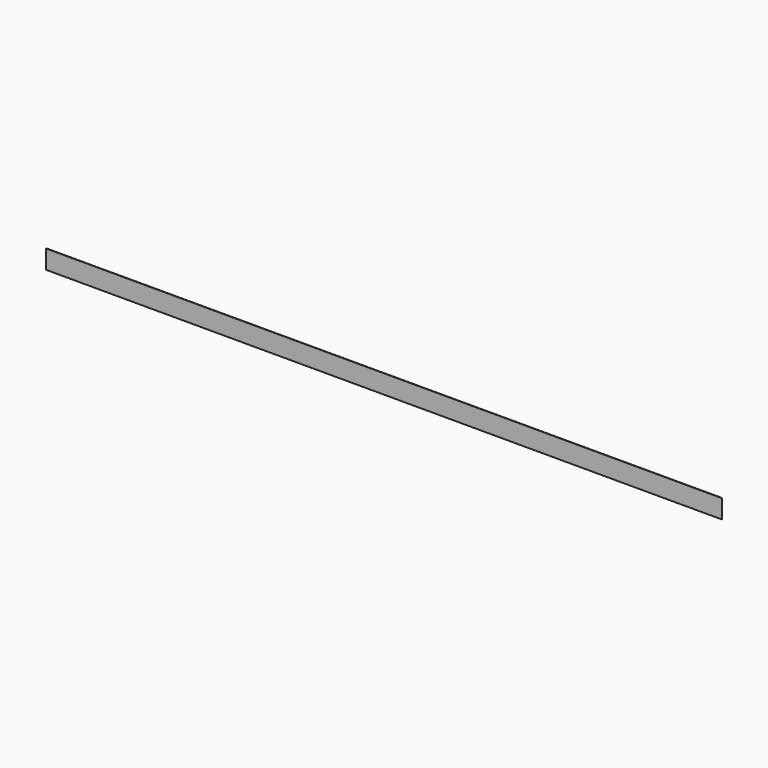
from build123d import *

# Parameters (mm, degrees)
F1_DEPTH = 914.4
F3_DEPTH = 76.2


# Not quite as in the source:
# - a pattern or mirror of a feature is missing from the dataset's text; its kind, count and spacing are read off the source's solid


with BuildPart() as f1:
    # F0 (on Right) → F1 (new body, symmetric)
    with BuildSketch(Plane.YZ):
        with BuildLine():
            Line((-50.8, 0), (0, 0))
            ThreePointArc((0, 0), (-0.9299359697, 2.2450640303), (-3.175, 3.175))
            Line((-3.175, 3.175), (-47.625, 3.175))
            Line((-47.625, 3.175), (-47.625, 47.625))
            ThreePointArc((-47.625, 47.625), (-48.5549359697, 49.8700640303), (-50.8, 50.8))
            Line((-50.8, 50.8), (-50.8, 0))
        make_face()
    extrude(amount=F1_DEPTH, both=True)

    # F2 (on face) → F3 (cut)
    with BuildSketch(Plane(origin=(0, 0, 0), x_dir=(1, 0, 0), z_dir=(0, 0, -1))):
        Polygon((914.4, 50.8), (863.6, 0), (914.4, 0), align=None)
    f3 = extrude(amount=-F3_DEPTH, mode=Mode.SUBTRACT)

    # F3_copies: F3 across plane
    add(f3.mirror(Plane(origin=(0, 0, 0), x_dir=(0, 0, -1), z_dir=(-1, 0, 0))), mode=Mode.SUBTRACT)


solid = f1.part
